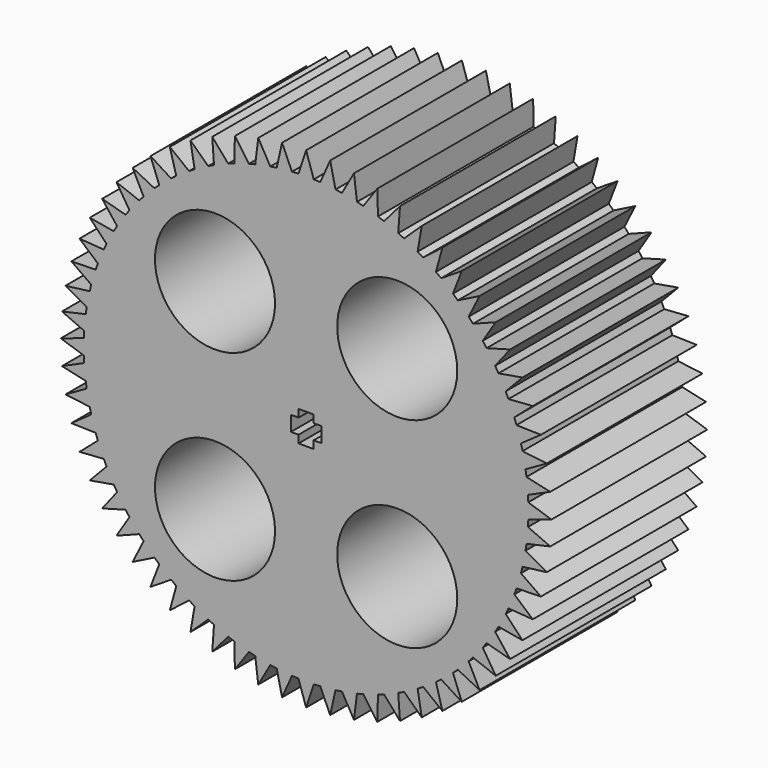
from build123d import *

# Parameters (mm, degrees)
F0_R     = 7.8312391684
F1_DEPTH = 7.0000114
F2_DEPTH = 25.4


with BuildPart() as f1:
    # F0 (on Front) → F1 (new body)
    with BuildSketch(Plane.XZ):
        with BuildLine():
            ThreePointArc((-1.00000054, 28.9827594773), (0, 29.000006), (1.00000054, 28.9827594773))
            Line((1.00000054, 28.9827594773), (0, 32))
            Line((0, 32), (-1.00000054, 28.9827594773))
        make_face()
        with BuildLine():
            ThreePointArc((1.8456219388, 28.9412167619), (2.8424976577, 28.8603630446), (3.8359924669, 28.7451823754))
            Line((3.8359924669, 28.7451823754), (3.1365484905, 31.8459112535))
            Line((3.1365484905, 31.8459112535), (1.8456219388, 28.9412167619))
        make_face()
        with BuildLine():
            ThreePointArc((4.6734700693, 28.6209543082), (5.657620509, 28.4427790164), (6.6350416894, 28.2307734535))
            Line((6.6350416894, 28.2307734535), (6.2428903045, 31.3851289729))
            Line((6.2428903045, 31.3851289729), (4.6734700693, 28.6209543082))
        make_face()
        with BuildLine():
            ThreePointArc((7.4563101283, 28.0250564187), (8.4182573821, 27.7512754779), (9.3701918333, 27.4444867507))
            Line((9.3701918333, 27.4444867507), (9.2891096721, 30.6220907434))
            Line((9.2891096721, 30.6220907434), (7.4563101283, 28.0250564187))
        make_face()
        with BuildLine():
            ThreePointArc((10.1673418448, 27.1592619158), (11.0978218347, 26.7925119861), (12.0151019076, 26.3938946378))
            Line((12.0151019076, 26.3938946378), (12.2458698357, 29.5641450404))
            Line((12.2458698357, 29.5641450404), (10.1673418448, 27.1592619158))
        make_face()
        with BuildLine():
            ThreePointArc((12.7804565012, 26.0319088739), (13.6705081963, 25.5757219576), (14.5442999824, 25.0891148912))
            Line((14.5442999824, 25.0891148912), (15.0846955784, 28.2214804591))
            Line((15.0846955784, 28.2214804591), (12.7804565012, 26.0319088739))
        make_face()
        with BuildLine():
            Line((28.9827594773, -1.00000054), (28.9827594773, 1.00000054))
            ThreePointArc((28.9827594773, 1.00000054), (28.9650742227, 1.4229628499), (28.9412167619, 1.8456219388))
            Line((28.9412167619, 1.8456219388), (28.7451823754, 3.8359924669))
            ThreePointArc((28.7451823754, 3.8359924669), (28.686124724, 4.2551846396), (28.6209543082, 4.6734700693))
            Line((28.6209543082, 4.6734700693), (28.2307734535, 6.6350416894))
            ThreePointArc((28.2307734535, 6.6350416894), (28.1309121628, 7.0464266751), (28.0250564187, 7.4563101283))
            Line((28.0250564187, 7.4563101283), (27.4444867507, 9.3701918333))
            ThreePointArc((27.4444867507, 9.3701918333), (27.3047835396, 9.7698077697), (27.1592619158, 10.1673418448))
            Line((27.1592619158, 10.1673418448), (26.3938946378, 12.0151019076))
            ThreePointArc((26.3938946378, 12.0151019076), (26.2156949245, 12.3991002748), (26.0319088739, 12.7804565012))
            Line((26.0319088739, 12.7804565012), (25.0891148912, 14.5442999824))
            ThreePointArc((25.0891148912, 14.5442999824), (24.8741348364, 14.9089826662), (24.6538543191, 15.2704883751))
            Line((24.6538543191, 15.2704883751), (23.542713253, 16.9334284977))
            ThreePointArc((23.542713253, 16.9334284977), (23.2930232322, 17.2752834045), (23.03836967, 17.6134570982))
            Line((23.03836967, 17.6134570982), (21.7695824165, 19.1594788397))
            ThreePointArc((21.7695824165, 19.1594788397), (21.487587081, 19.4752137199), (21.2010129269, 19.7867986009))
            Line((21.2010129269, 19.7867986009), (19.7867986009, 21.2010129269))
            ThreePointArc((19.7867986009, 21.2010129269), (19.4752137199, 21.487587081), (19.1594788397, 21.7695824165))
            Line((19.1594788397, 21.7695824165), (17.6134570982, 23.03836967))
            ThreePointArc((17.6134570982, 23.03836967), (17.2752834045, 23.2930232322), (16.9334284977, 23.542713253))
            Line((16.9334284977, 23.542713253), (15.2704883751, 24.6538543191))
            ThreePointArc((15.2704883751, 24.6538543191), (14.9089826662, 24.8741348364), (14.5442999824, 25.0891148912))
            Line((14.5442999824, 25.0891148912), (12.7804565012, 26.0319088739))
            ThreePointArc((12.7804565012, 26.0319088739), (12.3991002748, 26.2156949245), (12.0151019076, 26.3938946378))
            Line((12.0151019076, 26.3938946378), (10.1673418448, 27.1592619158))
            ThreePointArc((10.1673418448, 27.1592619158), (9.7698077697, 27.3047835396), (9.3701918333, 27.4444867507))
            Line((9.3701918333, 27.4444867507), (7.4563101283, 28.0250564187))
            ThreePointArc((7.4563101283, 28.0250564187), (7.0464266751, 28.1309121628), (6.6350416894, 28.2307734535))
            Line((6.6350416894, 28.2307734535), (4.6734700693, 28.6209543082))
            ThreePointArc((4.6734700693, 28.6209543082), (4.2551846396, 28.686124724), (3.8359924669, 28.7451823754))
            Line((3.8359924669, 28.7451823754), (1.8456219388, 28.9412167619))
            ThreePointArc((1.8456219388, 28.9412167619), (1.4229628499, 28.9650742227), (1.00000054, 28.9827594773))
            Line((1.00000054, 28.9827594773), (-1.00000054, 28.9827594773))
            ThreePointArc((-1.00000054, 28.9827594773), (-1.4229628499, 28.9650742227), (-1.8456219388, 28.9412167619))
            Line((-1.8456219388, 28.9412167619), (-3.8359924669, 28.7451823754))
            ThreePointArc((-3.8359924669, 28.7451823754), (-4.2551846396, 28.686124724), (-4.6734700693, 28.6209543082))
            Line((-4.6734700693, 28.6209543082), (-6.6350416894, 28.2307734535))
            ThreePointArc((-6.6350416894, 28.2307734535), (-7.0464266751, 28.1309121628), (-7.4563101283, 28.0250564187))
            Line((-7.4563101283, 28.0250564187), (-9.3701918333, 27.4444867507))
            ThreePointArc((-9.3701918333, 27.4444867507), (-9.7698077697, 27.3047835396), (-10.1673418448, 27.1592619158))
            Line((-10.1673418448, 27.1592619158), (-12.0151019076, 26.3938946378))
            ThreePointArc((-12.0151019076, 26.3938946378), (-12.3991002748, 26.2156949245), (-12.7804565012, 26.0319088739))
            Line((-12.7804565012, 26.0319088739), (-14.5442999824, 25.0891148912))
            ThreePointArc((-14.5442999824, 25.0891148912), (-14.9089826662, 24.8741348364), (-15.2704883751, 24.6538543191))
            Line((-15.2704883751, 24.6538543191), (-16.9334284977, 23.542713253))
            ThreePointArc((-16.9334284977, 23.542713253), (-17.2752834045, 23.2930232322), (-17.6134570982, 23.03836967))
            Line((-17.6134570982, 23.03836967), (-19.1594788397, 21.7695824165))
            ThreePointArc((-19.1594788397, 21.7695824165), (-19.4752137199, 21.487587081), (-19.7867986009, 21.2010129269))
            Line((-19.7867986009, 21.2010129269), (-21.2010129269, 19.7867986009))
            ThreePointArc((-21.2010129269, 19.7867986009), (-21.487587081, 19.4752137199), (-21.7695824165, 19.1594788397))
            Line((-21.7695824165, 19.1594788397), (-23.03836967, 17.6134570982))
            ThreePointArc((-23.03836967, 17.6134570982), (-23.2930232322, 17.2752834045), (-23.542713253, 16.9334284977))
            Line((-23.542713253, 16.9334284977), (-24.6538543191, 15.2704883751))
            ThreePointArc((-24.6538543191, 15.2704883751), (-24.8741348364, 14.9089826662), (-25.0891148912, 14.5442999824))
            Line((-25.0891148912, 14.5442999824), (-26.0319088739, 12.7804565012))
            ThreePointArc((-26.0319088739, 12.7804565012), (-26.2156949245, 12.3991002748), (-26.3938946378, 12.0151019076))
            Line((-26.3938946378, 12.0151019076), (-27.1592619158, 10.1673418448))
            ThreePointArc((-27.1592619158, 10.1673418448), (-27.3047835396, 9.7698077697), (-27.4444867507, 9.3701918333))
            Line((-27.4444867507, 9.3701918333), (-28.0250564187, 7.4563101283))
            ThreePointArc((-28.0250564187, 7.4563101283), (-28.1309121628, 7.0464266751), (-28.2307734535, 6.6350416894))
            Line((-28.2307734535, 6.6350416894), (-28.6209543082, 4.6734700693))
            ThreePointArc((-28.6209543082, 4.6734700693), (-28.686124724, 4.2551846396), (-28.7451823754, 3.8359924669))
            Line((-28.7451823754, 3.8359924669), (-28.9412167619, 1.8456219388))
            ThreePointArc((-28.9412167619, 1.8456219388), (-28.9650742227, 1.4229628499), (-28.9827594773, 1.00000054))
            Line((-28.9827594773, 1.00000054), (-28.9827594773, -1.00000054))
            ThreePointArc((-28.9827594773, -1.00000054), (-28.9650742227, -1.4229628499), (-28.9412167619, -1.8456219388))
            Line((-28.9412167619, -1.8456219388), (-28.7451823754, -3.8359924669))
            ThreePointArc((-28.7451823754, -3.8359924669), (-28.686124724, -4.2551846396), (-28.6209543082, -4.6734700693))
            Line((-28.6209543082, -4.6734700693), (-28.2307734535, -6.6350416894))
            ThreePointArc((-28.2307734535, -6.6350416894), (-28.1309121628, -7.0464266751), (-28.0250564187, -7.4563101283))
            Line((-28.0250564187, -7.4563101283), (-27.4444867507, -9.3701918333))
            ThreePointArc((-27.4444867507, -9.3701918333), (-27.3047835396, -9.7698077697), (-27.1592619158, -10.1673418448))
            Line((-27.1592619158, -10.1673418448), (-26.3938946378, -12.0151019076))
            ThreePointArc((-26.3938946378, -12.0151019076), (-26.2156949245, -12.3991002748), (-26.0319088739, -12.7804565012))
            Line((-26.0319088739, -12.7804565012), (-25.0891148912, -14.5442999824))
            ThreePointArc((-25.0891148912, -14.5442999824), (-24.8741348364, -14.9089826662), (-24.6538543191, -15.2704883751))
            Line((-24.6538543191, -15.2704883751), (-23.542713253, -16.9334284977))
            ThreePointArc((-23.542713253, -16.9334284977), (-23.2930232322, -17.2752834045), (-23.03836967, -17.6134570982))
            Line((-23.03836967, -17.6134570982), (-21.7695824165, -19.1594788397))
            ThreePointArc((-21.7695824165, -19.1594788397), (-21.487587081, -19.4752137199), (-21.2010129269, -19.7867986009))
            Line((-21.2010129269, -19.7867986009), (-19.7867986009, -21.2010129269))
            ThreePointArc((-19.7867986009, -21.2010129269), (-19.4752137199, -21.487587081), (-19.1594788397, -21.7695824165))
            Line((-19.1594788397, -21.7695824165), (-17.6134570982, -23.03836967))
            ThreePointArc((-17.6134570982, -23.03836967), (-17.2752834045, -23.2930232322), (-16.9334284977, -23.542713253))
            Line((-16.9334284977, -23.542713253), (-15.2704883751, -24.6538543191))
            ThreePointArc((-15.2704883751, -24.6538543191), (-14.9089826662, -24.8741348364), (-14.5442999824, -25.0891148912))
            Line((-14.5442999824, -25.0891148912), (-12.7804565012, -26.0319088739))
            ThreePointArc((-12.7804565012, -26.0319088739), (-12.3991002748, -26.2156949245), (-12.0151019076, -26.3938946378))
            Line((-12.0151019076, -26.3938946378), (-10.1673418448, -27.1592619158))
            ThreePointArc((-10.1673418448, -27.1592619158), (-9.7698077697, -27.3047835396), (-9.3701918333, -27.4444867507))
            Line((-9.3701918333, -27.4444867507), (-7.4563101283, -28.0250564187))
            ThreePointArc((-7.4563101283, -28.0250564187), (-7.0464266751, -28.1309121628), (-6.6350416894, -28.2307734535))
            Line((-6.6350416894, -28.2307734535), (-4.6734700693, -28.6209543082))
            ThreePointArc((-4.6734700693, -28.6209543082), (-4.2551846396, -28.686124724), (-3.8359924669, -28.7451823754))
            Line((-3.8359924669, -28.7451823754), (-1.8456219388, -28.9412167619))
            ThreePointArc((-1.8456219388, -28.9412167619), (-1.4229628499, -28.9650742227), (-1.00000054, -28.9827594773))
            Line((-1.00000054, -28.9827594773), (1.00000054, -28.9827594773))
            ThreePointArc((1.00000054, -28.9827594773), (1.4229628499, -28.9650742227), (1.8456219388, -28.9412167619))
            Line((1.8456219388, -28.9412167619), (3.8359924669, -28.7451823754))
            ThreePointArc((3.8359924669, -28.7451823754), (4.2551846396, -28.686124724), (4.6734700693, -28.6209543082))
            Line((4.6734700693, -28.6209543082), (6.6350416894, -28.2307734535))
            ThreePointArc((6.6350416894, -28.2307734535), (7.0464266751, -28.1309121628), (7.4563101283, -28.0250564187))
            Line((7.4563101283, -28.0250564187), (9.3701918333, -27.4444867507))
            ThreePointArc((9.3701918333, -27.4444867507), (9.7698077697, -27.3047835396), (10.1673418448, -27.1592619158))
            Line((10.1673418448, -27.1592619158), (12.0151019076, -26.3938946378))
            ThreePointArc((12.0151019076, -26.3938946378), (12.3991002748, -26.2156949245), (12.7804565012, -26.0319088739))
            Line((12.7804565012, -26.0319088739), (14.5442999824, -25.0891148912))
            ThreePointArc((14.5442999824, -25.0891148912), (14.9089826662, -24.8741348364), (15.2704883751, -24.6538543191))
            Line((15.2704883751, -24.6538543191), (16.9334284977, -23.542713253))
            ThreePointArc((16.9334284977, -23.542713253), (17.2752834045, -23.2930232322), (17.6134570982, -23.03836967))
            Line((17.6134570982, -23.03836967), (19.1594788397, -21.7695824165))
            ThreePointArc((19.1594788397, -21.7695824165), (19.4752137199, -21.487587081), (19.7867986009, -21.2010129269))
            Line((19.7867986009, -21.2010129269), (21.2010129269, -19.7867986009))
            ThreePointArc((21.2010129269, -19.7867986009), (21.487587081, -19.4752137199), (21.7695824165, -19.1594788397))
            Line((21.7695824165, -19.1594788397), (23.03836967, -17.6134570982))
            ThreePointArc((23.03836967, -17.6134570982), (23.2930232322, -17.2752834045), (23.542713253, -16.9334284977))
            Line((23.542713253, -16.9334284977), (24.6538543191, -15.2704883751))
            ThreePointArc((24.6538543191, -15.2704883751), (24.8741348364, -14.9089826662), (25.0891148912, -14.5442999824))
            Line((25.0891148912, -14.5442999824), (26.0319088739, -12.7804565012))
            ThreePointArc((26.0319088739, -12.7804565012), (26.2156949245, -12.3991002748), (26.3938946378, -12.0151019076))
            Line((26.3938946378, -12.0151019076), (27.1592619158, -10.1673418448))
            ThreePointArc((27.1592619158, -10.1673418448), (27.3047835396, -9.7698077697), (27.4444867507, -9.3701918333))
            Line((27.4444867507, -9.3701918333), (28.0250564187, -7.4563101283))
            ThreePointArc((28.0250564187, -7.4563101283), (28.1309121628, -7.0464266751), (28.2307734535, -6.6350416894))
            Line((28.2307734535, -6.6350416894), (28.6209543082, -4.6734700693))
            ThreePointArc((28.6209543082, -4.6734700693), (28.686124724, -4.2551846396), (28.7451823754, -3.8359924669))
            Line((28.7451823754, -3.8359924669), (28.9412167619, -1.8456219388))
            ThreePointArc((28.9412167619, -1.8456219388), (28.9650742227, -1.4229628499), (28.9827594773, -1.00000054))
        make_face()
        with Locations((-11.8841798976, -13.0854817107)):
            Circle(F0_R, mode=Mode.SUBTRACT)
        with Locations((11.8841798976, -13.0854817107)):
            Circle(F0_R, mode=Mode.SUBTRACT)
        with Locations((-11.8841798976, 13.0854817107)):
            Circle(F0_R, mode=Mode.SUBTRACT)
        Polygon((-0.98349054, 0.98349054), (-0.98349054, 1.98349108), (0.98349054, 1.98349108), (0.98349054, 0.98349054), (1.98349108, 0.98349054), (1.98349108, -0.98349054), (0.98349054, -0.98349054), (0.98349054, -1.98349108), (-0.98349054, -1.98349108), (-0.98349054, -0.98349054), (-1.98349108, -0.98349054), (-1.98349108, 0.98349054), align=None, mode=Mode.SUBTRACT)
        with Locations((11.8841798976, 13.0854817107)):
            Circle(F0_R, mode=Mode.SUBTRACT)
        with BuildLine():
            ThreePointArc((15.2704883751, 24.6538543191), (16.111540091, 24.1126237456), (16.9334284977, 23.542713253))
            Line((16.9334284977, 23.542713253), (17.7782474566, 26.6070275937))
            Line((17.7782474566, 26.6070275937), (15.2704883751, 24.6538543191))
        make_face()
        with BuildLine():
            ThreePointArc((17.6134570982, 23.03836967), (18.3974090471, 22.4173077856), (19.1594788397, 21.7695824165))
            Line((19.1594788397, 21.7695824165), (20.3005850932, 24.7363345076))
            Line((20.3005850932, 24.7363345076), (17.6134570982, 23.03836967))
        make_face()
        with BuildLine():
            ThreePointArc((19.7867986009, 21.2010129269), (20.5061008971, 20.5061008971), (21.2010129269, 19.7867986009))
            Line((21.2010129269, 19.7867986009), (22.627416998, 22.627416998))
            Line((22.627416998, 22.627416998), (19.7867986009, 21.2010129269))
        make_face()
        with BuildLine():
            ThreePointArc((21.7695824165, 19.1594788397), (22.4173077856, 18.3974090471), (23.03836967, 17.6134570982))
            Line((23.03836967, 17.6134570982), (24.7363345076, 20.3005850932))
            Line((24.7363345076, 20.3005850932), (21.7695824165, 19.1594788397))
        make_face()
        with BuildLine():
            ThreePointArc((23.542713253, 16.9334284977), (24.1126237456, 16.111540091), (24.6538543191, 15.2704883751))
            Line((24.6538543191, 15.2704883751), (26.6070275937, 17.7782474566))
            Line((26.6070275937, 17.7782474566), (23.542713253, 16.9334284977))
        make_face()
        with BuildLine():
            ThreePointArc((25.0891148912, 14.5442999824), (25.5757219576, 13.6705081963), (26.0319088739, 12.7804565012))
            Line((26.0319088739, 12.7804565012), (28.2214804591, 15.0846955784))
            Line((28.2214804591, 15.0846955784), (25.0891148912, 14.5442999824))
        make_face()
        with BuildLine():
            ThreePointArc((26.3938946378, 12.0151019076), (26.7925119861, 11.0978218347), (27.1592619158, 10.1673418448))
            Line((27.1592619158, 10.1673418448), (29.5641450404, 12.2458698357))
            Line((29.5641450404, 12.2458698357), (26.3938946378, 12.0151019076))
        make_face()
        with BuildLine():
            ThreePointArc((27.4444867507, 9.3701918333), (27.7512754779, 8.4182573821), (28.0250564187, 7.4563101283))
            Line((28.0250564187, 7.4563101283), (30.6220907434, 9.2891096721))
            Line((30.6220907434, 9.2891096721), (27.4444867507, 9.3701918333))
        make_face()
        with BuildLine():
            ThreePointArc((28.2307734535, 6.6350416894), (28.4427790164, 5.657620509), (28.6209543082, 4.6734700693))
            Line((28.6209543082, 4.6734700693), (31.3851289729, 6.2428903045))
            Line((31.3851289729, 6.2428903045), (28.2307734535, 6.6350416894))
        make_face()
        with BuildLine():
            ThreePointArc((28.7451823754, 3.8359924669), (28.8603630446, 2.8424976577), (28.9412167619, 1.8456219388))
            Line((28.9412167619, 1.8456219388), (31.8459112535, 3.1365484905))
            Line((31.8459112535, 3.1365484905), (28.7451823754, 3.8359924669))
        make_face()
        with BuildLine():
            ThreePointArc((28.9827594773, 1.00000054), (28.9956940488, 0.5000746251), (29.000006, 0))
            ThreePointArc((29.000006, 0), (28.9956940488, -0.5000746251), (28.9827594773, -1.00000054))
            Line((28.9827594773, -1.00000054), (32, 0))
            Line((32, 0), (28.9827594773, 1.00000054))
        make_face()
        with BuildLine():
            Line((31.8459112535, -3.1365484905), (28.9412167619, -1.8456219388))
            ThreePointArc((28.9412167619, -1.8456219388), (28.8603630446, -2.8424976577), (28.7451823754, -3.8359924669))
            Line((28.7451823754, -3.8359924669), (31.8459112535, -3.1365484905))
        make_face()
        with BuildLine():
            Line((31.3851289729, -6.2428903045), (28.6209543082, -4.6734700693))
            ThreePointArc((28.6209543082, -4.6734700693), (28.4427790164, -5.657620509), (28.2307734535, -6.6350416894))
            Line((28.2307734535, -6.6350416894), (31.3851289729, -6.2428903045))
        make_face()
        with BuildLine():
            Line((30.6220907434, -9.2891096721), (28.0250564187, -7.4563101283))
            ThreePointArc((28.0250564187, -7.4563101283), (27.7512754779, -8.4182573821), (27.4444867507, -9.3701918333))
            Line((27.4444867507, -9.3701918333), (30.6220907434, -9.2891096721))
        make_face()
        with BuildLine():
            Line((29.5641450404, -12.2458698357), (27.1592619158, -10.1673418448))
            ThreePointArc((27.1592619158, -10.1673418448), (26.7925119861, -11.0978218347), (26.3938946378, -12.0151019076))
            Line((26.3938946378, -12.0151019076), (29.5641450404, -12.2458698357))
        make_face()
        with BuildLine():
            Line((26.6070275937, -17.7782474566), (24.6538543191, -15.2704883751))
            ThreePointArc((24.6538543191, -15.2704883751), (24.1126237456, -16.111540091), (23.542713253, -16.9334284977))
            Line((23.542713253, -16.9334284977), (26.6070275937, -17.7782474566))
        make_face()
        with BuildLine():
            Line((28.2214804591, -15.0846955784), (26.0319088739, -12.7804565012))
            ThreePointArc((26.0319088739, -12.7804565012), (25.5757219576, -13.6705081963), (25.0891148912, -14.5442999824))
            Line((25.0891148912, -14.5442999824), (28.2214804591, -15.0846955784))
        make_face()
        with BuildLine():
            Line((24.7363345076, -20.3005850932), (23.03836967, -17.6134570982))
            ThreePointArc((23.03836967, -17.6134570982), (22.4173077856, -18.3974090471), (21.7695824165, -19.1594788397))
            Line((21.7695824165, -19.1594788397), (24.7363345076, -20.3005850932))
        make_face()
        with BuildLine():
            Line((22.627416998, -22.627416998), (21.2010129269, -19.7867986009))
            ThreePointArc((21.2010129269, -19.7867986009), (20.5061008971, -20.5061008971), (19.7867986009, -21.2010129269))
            Line((19.7867986009, -21.2010129269), (22.627416998, -22.627416998))
        make_face()
        with BuildLine():
            Line((20.3005850932, -24.7363345076), (19.1594788397, -21.7695824165))
            ThreePointArc((19.1594788397, -21.7695824165), (18.3974090471, -22.4173077856), (17.6134570982, -23.03836967))
            Line((17.6134570982, -23.03836967), (20.3005850932, -24.7363345076))
        make_face()
        with BuildLine():
            Line((17.7782474566, -26.6070275937), (16.9334284977, -23.542713253))
            ThreePointArc((16.9334284977, -23.542713253), (16.111540091, -24.1126237456), (15.2704883751, -24.6538543191))
            Line((15.2704883751, -24.6538543191), (17.7782474566, -26.6070275937))
        make_face()
        with BuildLine():
            Line((15.0846955784, -28.2214804591), (14.5442999824, -25.0891148912))
            ThreePointArc((14.5442999824, -25.0891148912), (13.6705081963, -25.5757219576), (12.7804565012, -26.0319088739))
            Line((12.7804565012, -26.0319088739), (15.0846955784, -28.2214804591))
        make_face()
        with BuildLine():
            Line((12.2458698357, -29.5641450404), (12.0151019076, -26.3938946378))
            ThreePointArc((12.0151019076, -26.3938946378), (11.0978218347, -26.7925119861), (10.1673418448, -27.1592619158))
            Line((10.1673418448, -27.1592619158), (12.2458698357, -29.5641450404))
        make_face()
        with BuildLine():
            Line((9.2891096721, -30.6220907434), (9.3701918333, -27.4444867507))
            ThreePointArc((9.3701918333, -27.4444867507), (8.4182573821, -27.7512754779), (7.4563101283, -28.0250564187))
            Line((7.4563101283, -28.0250564187), (9.2891096721, -30.6220907434))
        make_face()
        with BuildLine():
            Line((6.2428903045, -31.3851289729), (6.6350416894, -28.2307734535))
            ThreePointArc((6.6350416894, -28.2307734535), (5.657620509, -28.4427790164), (4.6734700693, -28.6209543082))
            Line((4.6734700693, -28.6209543082), (6.2428903045, -31.3851289729))
        make_face()
        with BuildLine():
            Line((3.1365484905, -31.8459112535), (3.8359924669, -28.7451823754))
            ThreePointArc((3.8359924669, -28.7451823754), (2.8424976577, -28.8603630446), (1.8456219388, -28.9412167619))
            Line((1.8456219388, -28.9412167619), (3.1365484905, -31.8459112535))
        make_face()
        with BuildLine():
            Line((0, -32), (1.00000054, -28.9827594773))
            ThreePointArc((1.00000054, -28.9827594773), (0, -29.000006), (-1.00000054, -28.9827594773))
            Line((-1.00000054, -28.9827594773), (0, -32))
        make_face()
        with BuildLine():
            Line((-3.1365484905, -31.8459112535), (-1.8456219388, -28.9412167619))
            ThreePointArc((-1.8456219388, -28.9412167619), (-2.8424976577, -28.8603630446), (-3.8359924669, -28.7451823754))
            Line((-3.8359924669, -28.7451823754), (-3.1365484905, -31.8459112535))
        make_face()
        with BuildLine():
            Line((-6.2428903045, -31.3851289729), (-4.6734700693, -28.6209543082))
            ThreePointArc((-4.6734700693, -28.6209543082), (-5.657620509, -28.4427790164), (-6.6350416894, -28.2307734535))
            Line((-6.6350416894, -28.2307734535), (-6.2428903045, -31.3851289729))
        make_face()
        with BuildLine():
            Line((-9.2891096721, -30.6220907434), (-7.4563101283, -28.0250564187))
            ThreePointArc((-7.4563101283, -28.0250564187), (-8.4182573821, -27.7512754779), (-9.3701918333, -27.4444867507))
            Line((-9.3701918333, -27.4444867507), (-9.2891096721, -30.6220907434))
        make_face()
        with BuildLine():
            Line((-12.2458698357, -29.5641450404), (-10.1673418448, -27.1592619158))
            ThreePointArc((-10.1673418448, -27.1592619158), (-11.0978218347, -26.7925119861), (-12.0151019076, -26.3938946378))
            Line((-12.0151019076, -26.3938946378), (-12.2458698357, -29.5641450404))
        make_face()
        with BuildLine():
            Line((-15.0846955784, -28.2214804591), (-12.7804565012, -26.0319088739))
            ThreePointArc((-12.7804565012, -26.0319088739), (-13.6705081963, -25.5757219576), (-14.5442999824, -25.0891148912))
            Line((-14.5442999824, -25.0891148912), (-15.0846955784, -28.2214804591))
        make_face()
        with BuildLine():
            Line((-17.7782474566, -26.6070275937), (-15.2704883751, -24.6538543191))
            ThreePointArc((-15.2704883751, -24.6538543191), (-16.111540091, -24.1126237456), (-16.9334284977, -23.542713253))
            Line((-16.9334284977, -23.542713253), (-17.7782474566, -26.6070275937))
        make_face()
        with BuildLine():
            Line((-20.3005850932, -24.7363345076), (-17.6134570982, -23.03836967))
            ThreePointArc((-17.6134570982, -23.03836967), (-18.3974090471, -22.4173077856), (-19.1594788397, -21.7695824165))
            Line((-19.1594788397, -21.7695824165), (-20.3005850932, -24.7363345076))
        make_face()
        with BuildLine():
            Line((-22.627416998, -22.627416998), (-19.7867986009, -21.2010129269))
            ThreePointArc((-19.7867986009, -21.2010129269), (-20.5061008971, -20.5061008971), (-21.2010129269, -19.7867986009))
            Line((-21.2010129269, -19.7867986009), (-22.627416998, -22.627416998))
        make_face()
        with BuildLine():
            Line((-24.7363345076, -20.3005850932), (-21.7695824165, -19.1594788397))
            ThreePointArc((-21.7695824165, -19.1594788397), (-22.4173077856, -18.3974090471), (-23.03836967, -17.6134570982))
            Line((-23.03836967, -17.6134570982), (-24.7363345076, -20.3005850932))
        make_face()
        with BuildLine():
            Line((-26.6070275937, -17.7782474566), (-23.542713253, -16.9334284977))
            ThreePointArc((-23.542713253, -16.9334284977), (-24.1126237456, -16.111540091), (-24.6538543191, -15.2704883751))
            Line((-24.6538543191, -15.2704883751), (-26.6070275937, -17.7782474566))
        make_face()
        with BuildLine():
            Line((-28.2214804591, -15.0846955784), (-25.0891148912, -14.5442999824))
            ThreePointArc((-25.0891148912, -14.5442999824), (-25.5757219576, -13.6705081963), (-26.0319088739, -12.7804565012))
            Line((-26.0319088739, -12.7804565012), (-28.2214804591, -15.0846955784))
        make_face()
        with BuildLine():
            Line((-29.5641450404, -12.2458698357), (-26.3938946378, -12.0151019076))
            ThreePointArc((-26.3938946378, -12.0151019076), (-26.7925119861, -11.0978218347), (-27.1592619158, -10.1673418448))
            Line((-27.1592619158, -10.1673418448), (-29.5641450404, -12.2458698357))
        make_face()
        with BuildLine():
            Line((-30.6220907434, -9.2891096721), (-27.4444867507, -9.3701918333))
            ThreePointArc((-27.4444867507, -9.3701918333), (-27.7512754779, -8.4182573821), (-28.0250564187, -7.4563101283))
            Line((-28.0250564187, -7.4563101283), (-30.6220907434, -9.2891096721))
        make_face()
        with BuildLine():
            Line((-31.3851289729, -6.2428903045), (-28.2307734535, -6.6350416894))
            ThreePointArc((-28.2307734535, -6.6350416894), (-28.4427790164, -5.657620509), (-28.6209543082, -4.6734700693))
            Line((-28.6209543082, -4.6734700693), (-31.3851289729, -6.2428903045))
        make_face()
        with BuildLine():
            Line((-31.8459112535, -3.1365484905), (-28.7451823754, -3.8359924669))
            ThreePointArc((-28.7451823754, -3.8359924669), (-28.8603630446, -2.8424976577), (-28.9412167619, -1.8456219388))
            Line((-28.9412167619, -1.8456219388), (-31.8459112535, -3.1365484905))
        make_face()
        with BuildLine():
            ThreePointArc((-28.9412167619, 1.8456219388), (-28.8603630446, 2.8424976577), (-28.7451823754, 3.8359924669))
            Line((-28.7451823754, 3.8359924669), (-31.8459112535, 3.1365484905))
            Line((-31.8459112535, 3.1365484905), (-28.9412167619, 1.8456219388))
        make_face()
        with BuildLine():
            ThreePointArc((-28.9827594773, -1.00000054), (-29.000006, 0), (-28.9827594773, 1.00000054))
            Line((-28.9827594773, 1.00000054), (-32, 0))
            Line((-32, 0), (-28.9827594773, -1.00000054))
        make_face()
        with BuildLine():
            ThreePointArc((-28.6209543082, 4.6734700693), (-28.4427790164, 5.657620509), (-28.2307734535, 6.6350416894))
            Line((-28.2307734535, 6.6350416894), (-31.3851289729, 6.2428903045))
            Line((-31.3851289729, 6.2428903045), (-28.6209543082, 4.6734700693))
        make_face()
        with BuildLine():
            ThreePointArc((-28.0250564187, 7.4563101283), (-27.7512754779, 8.4182573821), (-27.4444867507, 9.3701918333))
            Line((-27.4444867507, 9.3701918333), (-30.6220907434, 9.2891096721))
            Line((-30.6220907434, 9.2891096721), (-28.0250564187, 7.4563101283))
        make_face()
        with BuildLine():
            ThreePointArc((-27.1592619158, 10.1673418448), (-26.7925119861, 11.0978218347), (-26.3938946378, 12.0151019076))
            Line((-26.3938946378, 12.0151019076), (-29.5641450404, 12.2458698357))
            Line((-29.5641450404, 12.2458698357), (-27.1592619158, 10.1673418448))
        make_face()
        with BuildLine():
            ThreePointArc((-26.0319088739, 12.7804565012), (-25.5757219576, 13.6705081963), (-25.0891148912, 14.5442999824))
            Line((-25.0891148912, 14.5442999824), (-28.2214804591, 15.0846955784))
            Line((-28.2214804591, 15.0846955784), (-26.0319088739, 12.7804565012))
        make_face()
        with BuildLine():
            ThreePointArc((-24.6538543191, 15.2704883751), (-24.1126237456, 16.111540091), (-23.542713253, 16.9334284977))
            Line((-23.542713253, 16.9334284977), (-26.6070275937, 17.7782474566))
            Line((-26.6070275937, 17.7782474566), (-24.6538543191, 15.2704883751))
        make_face()
        with BuildLine():
            ThreePointArc((-23.03836967, 17.6134570982), (-22.4173077856, 18.3974090471), (-21.7695824165, 19.1594788397))
            Line((-21.7695824165, 19.1594788397), (-24.7363345076, 20.3005850932))
            Line((-24.7363345076, 20.3005850932), (-23.03836967, 17.6134570982))
        make_face()
        with BuildLine():
            ThreePointArc((-21.2010129269, 19.7867986009), (-20.5061008971, 20.5061008971), (-19.7867986009, 21.2010129269))
            Line((-19.7867986009, 21.2010129269), (-22.627416998, 22.627416998))
            Line((-22.627416998, 22.627416998), (-21.2010129269, 19.7867986009))
        make_face()
        with BuildLine():
            ThreePointArc((-19.1594788397, 21.7695824165), (-18.3974090471, 22.4173077856), (-17.6134570982, 23.03836967))
            Line((-17.6134570982, 23.03836967), (-20.3005850932, 24.7363345076))
            Line((-20.3005850932, 24.7363345076), (-19.1594788397, 21.7695824165))
        make_face()
        with BuildLine():
            ThreePointArc((-16.9334284977, 23.542713253), (-16.111540091, 24.1126237456), (-15.2704883751, 24.6538543191))
            Line((-15.2704883751, 24.6538543191), (-17.7782474566, 26.6070275937))
            Line((-17.7782474566, 26.6070275937), (-16.9334284977, 23.542713253))
        make_face()
        with BuildLine():
            ThreePointArc((-14.5442999824, 25.0891148912), (-13.6705081963, 25.5757219576), (-12.7804565012, 26.0319088739))
            Line((-12.7804565012, 26.0319088739), (-15.0846955784, 28.2214804591))
            Line((-15.0846955784, 28.2214804591), (-14.5442999824, 25.0891148912))
        make_face()
        with BuildLine():
            ThreePointArc((-12.0151019076, 26.3938946378), (-11.0978218347, 26.7925119861), (-10.1673418448, 27.1592619158))
            Line((-10.1673418448, 27.1592619158), (-12.2458698357, 29.5641450404))
            Line((-12.2458698357, 29.5641450404), (-12.0151019076, 26.3938946378))
        make_face()
        with BuildLine():
            ThreePointArc((-9.3701918333, 27.4444867507), (-8.4182573821, 27.7512754779), (-7.4563101283, 28.0250564187))
            Line((-7.4563101283, 28.0250564187), (-9.2891096721, 30.6220907434))
            Line((-9.2891096721, 30.6220907434), (-9.3701918333, 27.4444867507))
        make_face()
        with BuildLine():
            ThreePointArc((-6.6350416894, 28.2307734535), (-5.657620509, 28.4427790164), (-4.6734700693, 28.6209543082))
            Line((-4.6734700693, 28.6209543082), (-6.2428903045, 31.3851289729))
            Line((-6.2428903045, 31.3851289729), (-6.6350416894, 28.2307734535))
        make_face()
        with BuildLine():
            ThreePointArc((-3.8359924669, 28.7451823754), (-2.8424976577, 28.8603630446), (-1.8456219388, 28.9412167619))
            Line((-1.8456219388, 28.9412167619), (-3.1365484905, 31.8459112535))
            Line((-3.1365484905, 31.8459112535), (-3.8359924669, 28.7451823754))
        make_face()
    extrude(amount=F1_DEPTH)


with BuildPart() as f2:
    # F0 (on Front) → F2 (new body)
    with BuildSketch(Plane.XZ):
        with BuildLine():
            ThreePointArc((28.9827594773, -1.00000054), (28.9956940488, -0.5000746251), (29.000006, 0))
            ThreePointArc((29.000006, 0), (28.9956940488, 0.5000746251), (28.9827594773, 1.00000054))
            Line((28.9827594773, 1.00000054), (28.9827594773, -1.00000054))
        make_face()
        with BuildLine():
            ThreePointArc((28.9827594773, 1.00000054), (28.9956940488, 0.5000746251), (29.000006, 0))
            ThreePointArc((29.000006, 0), (28.9956940488, -0.5000746251), (28.9827594773, -1.00000054))
            Line((28.9827594773, -1.00000054), (32, 0))
            Line((32, 0), (28.9827594773, 1.00000054))
        make_face()
        with BuildLine():
            Line((28.9827594773, -1.00000054), (28.9827594773, 1.00000054))
            ThreePointArc((28.9827594773, 1.00000054), (28.9650742227, 1.4229628499), (28.9412167619, 1.8456219388))
            Line((28.9412167619, 1.8456219388), (28.7451823754, 3.8359924669))
            ThreePointArc((28.7451823754, 3.8359924669), (28.686124724, 4.2551846396), (28.6209543082, 4.6734700693))
            Line((28.6209543082, 4.6734700693), (28.2307734535, 6.6350416894))
            ThreePointArc((28.2307734535, 6.6350416894), (28.1309121628, 7.0464266751), (28.0250564187, 7.4563101283))
            Line((28.0250564187, 7.4563101283), (27.4444867507, 9.3701918333))
            ThreePointArc((27.4444867507, 9.3701918333), (27.3047835396, 9.7698077697), (27.1592619158, 10.1673418448))
            Line((27.1592619158, 10.1673418448), (26.3938946378, 12.0151019076))
            ThreePointArc((26.3938946378, 12.0151019076), (26.2156949245, 12.3991002748), (26.0319088739, 12.7804565012))
            Line((26.0319088739, 12.7804565012), (25.0891148912, 14.5442999824))
            ThreePointArc((25.0891148912, 14.5442999824), (24.8741348364, 14.9089826662), (24.6538543191, 15.2704883751))
            Line((24.6538543191, 15.2704883751), (23.542713253, 16.9334284977))
            ThreePointArc((23.542713253, 16.9334284977), (23.2930232322, 17.2752834045), (23.03836967, 17.6134570982))
            Line((23.03836967, 17.6134570982), (21.7695824165, 19.1594788397))
            ThreePointArc((21.7695824165, 19.1594788397), (21.487587081, 19.4752137199), (21.2010129269, 19.7867986009))
            Line((21.2010129269, 19.7867986009), (19.7867986009, 21.2010129269))
            ThreePointArc((19.7867986009, 21.2010129269), (19.4752137199, 21.487587081), (19.1594788397, 21.7695824165))
            Line((19.1594788397, 21.7695824165), (17.6134570982, 23.03836967))
            ThreePointArc((17.6134570982, 23.03836967), (17.2752834045, 23.2930232322), (16.9334284977, 23.542713253))
            Line((16.9334284977, 23.542713253), (15.2704883751, 24.6538543191))
            ThreePointArc((15.2704883751, 24.6538543191), (14.9089826662, 24.8741348364), (14.5442999824, 25.0891148912))
            Line((14.5442999824, 25.0891148912), (12.7804565012, 26.0319088739))
            ThreePointArc((12.7804565012, 26.0319088739), (12.3991002748, 26.2156949245), (12.0151019076, 26.3938946378))
            Line((12.0151019076, 26.3938946378), (10.1673418448, 27.1592619158))
            ThreePointArc((10.1673418448, 27.1592619158), (9.7698077697, 27.3047835396), (9.3701918333, 27.4444867507))
            Line((9.3701918333, 27.4444867507), (7.4563101283, 28.0250564187))
            ThreePointArc((7.4563101283, 28.0250564187), (7.0464266751, 28.1309121628), (6.6350416894, 28.2307734535))
            Line((6.6350416894, 28.2307734535), (4.6734700693, 28.6209543082))
            ThreePointArc((4.6734700693, 28.6209543082), (4.2551846396, 28.686124724), (3.8359924669, 28.7451823754))
            Line((3.8359924669, 28.7451823754), (1.8456219388, 28.9412167619))
            ThreePointArc((1.8456219388, 28.9412167619), (1.4229628499, 28.9650742227), (1.00000054, 28.9827594773))
            Line((1.00000054, 28.9827594773), (-1.00000054, 28.9827594773))
            ThreePointArc((-1.00000054, 28.9827594773), (-1.4229628499, 28.9650742227), (-1.8456219388, 28.9412167619))
            Line((-1.8456219388, 28.9412167619), (-3.8359924669, 28.7451823754))
            ThreePointArc((-3.8359924669, 28.7451823754), (-4.2551846396, 28.686124724), (-4.6734700693, 28.6209543082))
            Line((-4.6734700693, 28.6209543082), (-6.6350416894, 28.2307734535))
            ThreePointArc((-6.6350416894, 28.2307734535), (-7.0464266751, 28.1309121628), (-7.4563101283, 28.0250564187))
            Line((-7.4563101283, 28.0250564187), (-9.3701918333, 27.4444867507))
            ThreePointArc((-9.3701918333, 27.4444867507), (-9.7698077697, 27.3047835396), (-10.1673418448, 27.1592619158))
            Line((-10.1673418448, 27.1592619158), (-12.0151019076, 26.3938946378))
            ThreePointArc((-12.0151019076, 26.3938946378), (-12.3991002748, 26.2156949245), (-12.7804565012, 26.0319088739))
            Line((-12.7804565012, 26.0319088739), (-14.5442999824, 25.0891148912))
            ThreePointArc((-14.5442999824, 25.0891148912), (-14.9089826662, 24.8741348364), (-15.2704883751, 24.6538543191))
            Line((-15.2704883751, 24.6538543191), (-16.9334284977, 23.542713253))
            ThreePointArc((-16.9334284977, 23.542713253), (-17.2752834045, 23.2930232322), (-17.6134570982, 23.03836967))
            Line((-17.6134570982, 23.03836967), (-19.1594788397, 21.7695824165))
            ThreePointArc((-19.1594788397, 21.7695824165), (-19.4752137199, 21.487587081), (-19.7867986009, 21.2010129269))
            Line((-19.7867986009, 21.2010129269), (-21.2010129269, 19.7867986009))
            ThreePointArc((-21.2010129269, 19.7867986009), (-21.487587081, 19.4752137199), (-21.7695824165, 19.1594788397))
            Line((-21.7695824165, 19.1594788397), (-23.03836967, 17.6134570982))
            ThreePointArc((-23.03836967, 17.6134570982), (-23.2930232322, 17.2752834045), (-23.542713253, 16.9334284977))
            Line((-23.542713253, 16.9334284977), (-24.6538543191, 15.2704883751))
            ThreePointArc((-24.6538543191, 15.2704883751), (-24.8741348364, 14.9089826662), (-25.0891148912, 14.5442999824))
            Line((-25.0891148912, 14.5442999824), (-26.0319088739, 12.7804565012))
            ThreePointArc((-26.0319088739, 12.7804565012), (-26.2156949245, 12.3991002748), (-26.3938946378, 12.0151019076))
            Line((-26.3938946378, 12.0151019076), (-27.1592619158, 10.1673418448))
            ThreePointArc((-27.1592619158, 10.1673418448), (-27.3047835396, 9.7698077697), (-27.4444867507, 9.3701918333))
            Line((-27.4444867507, 9.3701918333), (-28.0250564187, 7.4563101283))
            ThreePointArc((-28.0250564187, 7.4563101283), (-28.1309121628, 7.0464266751), (-28.2307734535, 6.6350416894))
            Line((-28.2307734535, 6.6350416894), (-28.6209543082, 4.6734700693))
            ThreePointArc((-28.6209543082, 4.6734700693), (-28.686124724, 4.2551846396), (-28.7451823754, 3.8359924669))
            Line((-28.7451823754, 3.8359924669), (-28.9412167619, 1.8456219388))
            ThreePointArc((-28.9412167619, 1.8456219388), (-28.9650742227, 1.4229628499), (-28.9827594773, 1.00000054))
            Line((-28.9827594773, 1.00000054), (-28.9827594773, -1.00000054))
            ThreePointArc((-28.9827594773, -1.00000054), (-28.9650742227, -1.4229628499), (-28.9412167619, -1.8456219388))
            Line((-28.9412167619, -1.8456219388), (-28.7451823754, -3.8359924669))
            ThreePointArc((-28.7451823754, -3.8359924669), (-28.686124724, -4.2551846396), (-28.6209543082, -4.6734700693))
            Line((-28.6209543082, -4.6734700693), (-28.2307734535, -6.6350416894))
            ThreePointArc((-28.2307734535, -6.6350416894), (-28.1309121628, -7.0464266751), (-28.0250564187, -7.4563101283))
            Line((-28.0250564187, -7.4563101283), (-27.4444867507, -9.3701918333))
            ThreePointArc((-27.4444867507, -9.3701918333), (-27.3047835396, -9.7698077697), (-27.1592619158, -10.1673418448))
            Line((-27.1592619158, -10.1673418448), (-26.3938946378, -12.0151019076))
            ThreePointArc((-26.3938946378, -12.0151019076), (-26.2156949245, -12.3991002748), (-26.0319088739, -12.7804565012))
            Line((-26.0319088739, -12.7804565012), (-25.0891148912, -14.5442999824))
            ThreePointArc((-25.0891148912, -14.5442999824), (-24.8741348364, -14.9089826662), (-24.6538543191, -15.2704883751))
            Line((-24.6538543191, -15.2704883751), (-23.542713253, -16.9334284977))
            ThreePointArc((-23.542713253, -16.9334284977), (-23.2930232322, -17.2752834045), (-23.03836967, -17.6134570982))
            Line((-23.03836967, -17.6134570982), (-21.7695824165, -19.1594788397))
            ThreePointArc((-21.7695824165, -19.1594788397), (-21.487587081, -19.4752137199), (-21.2010129269, -19.7867986009))
            Line((-21.2010129269, -19.7867986009), (-19.7867986009, -21.2010129269))
            ThreePointArc((-19.7867986009, -21.2010129269), (-19.4752137199, -21.487587081), (-19.1594788397, -21.7695824165))
            Line((-19.1594788397, -21.7695824165), (-17.6134570982, -23.03836967))
            ThreePointArc((-17.6134570982, -23.03836967), (-17.2752834045, -23.2930232322), (-16.9334284977, -23.542713253))
            Line((-16.9334284977, -23.542713253), (-15.2704883751, -24.6538543191))
            ThreePointArc((-15.2704883751, -24.6538543191), (-14.9089826662, -24.8741348364), (-14.5442999824, -25.0891148912))
            Line((-14.5442999824, -25.0891148912), (-12.7804565012, -26.0319088739))
            ThreePointArc((-12.7804565012, -26.0319088739), (-12.3991002748, -26.2156949245), (-12.0151019076, -26.3938946378))
            Line((-12.0151019076, -26.3938946378), (-10.1673418448, -27.1592619158))
            ThreePointArc((-10.1673418448, -27.1592619158), (-9.7698077697, -27.3047835396), (-9.3701918333, -27.4444867507))
            Line((-9.3701918333, -27.4444867507), (-7.4563101283, -28.0250564187))
            ThreePointArc((-7.4563101283, -28.0250564187), (-7.0464266751, -28.1309121628), (-6.6350416894, -28.2307734535))
            Line((-6.6350416894, -28.2307734535), (-4.6734700693, -28.6209543082))
            ThreePointArc((-4.6734700693, -28.6209543082), (-4.2551846396, -28.686124724), (-3.8359924669, -28.7451823754))
            Line((-3.8359924669, -28.7451823754), (-1.8456219388, -28.9412167619))
            ThreePointArc((-1.8456219388, -28.9412167619), (-1.4229628499, -28.9650742227), (-1.00000054, -28.9827594773))
            Line((-1.00000054, -28.9827594773), (1.00000054, -28.9827594773))
            ThreePointArc((1.00000054, -28.9827594773), (1.4229628499, -28.9650742227), (1.8456219388, -28.9412167619))
            Line((1.8456219388, -28.9412167619), (3.8359924669, -28.7451823754))
            ThreePointArc((3.8359924669, -28.7451823754), (4.2551846396, -28.686124724), (4.6734700693, -28.6209543082))
            Line((4.6734700693, -28.6209543082), (6.6350416894, -28.2307734535))
            ThreePointArc((6.6350416894, -28.2307734535), (7.0464266751, -28.1309121628), (7.4563101283, -28.0250564187))
            Line((7.4563101283, -28.0250564187), (9.3701918333, -27.4444867507))
            ThreePointArc((9.3701918333, -27.4444867507), (9.7698077697, -27.3047835396), (10.1673418448, -27.1592619158))
            Line((10.1673418448, -27.1592619158), (12.0151019076, -26.3938946378))
            ThreePointArc((12.0151019076, -26.3938946378), (12.3991002748, -26.2156949245), (12.7804565012, -26.0319088739))
            Line((12.7804565012, -26.0319088739), (14.5442999824, -25.0891148912))
            ThreePointArc((14.5442999824, -25.0891148912), (14.9089826662, -24.8741348364), (15.2704883751, -24.6538543191))
            Line((15.2704883751, -24.6538543191), (16.9334284977, -23.542713253))
            ThreePointArc((16.9334284977, -23.542713253), (17.2752834045, -23.2930232322), (17.6134570982, -23.03836967))
            Line((17.6134570982, -23.03836967), (19.1594788397, -21.7695824165))
            ThreePointArc((19.1594788397, -21.7695824165), (19.4752137199, -21.487587081), (19.7867986009, -21.2010129269))
            Line((19.7867986009, -21.2010129269), (21.2010129269, -19.7867986009))
            ThreePointArc((21.2010129269, -19.7867986009), (21.487587081, -19.4752137199), (21.7695824165, -19.1594788397))
            Line((21.7695824165, -19.1594788397), (23.03836967, -17.6134570982))
            ThreePointArc((23.03836967, -17.6134570982), (23.2930232322, -17.2752834045), (23.542713253, -16.9334284977))
            Line((23.542713253, -16.9334284977), (24.6538543191, -15.2704883751))
            ThreePointArc((24.6538543191, -15.2704883751), (24.8741348364, -14.9089826662), (25.0891148912, -14.5442999824))
            Line((25.0891148912, -14.5442999824), (26.0319088739, -12.7804565012))
            ThreePointArc((26.0319088739, -12.7804565012), (26.2156949245, -12.3991002748), (26.3938946378, -12.0151019076))
            Line((26.3938946378, -12.0151019076), (27.1592619158, -10.1673418448))
            ThreePointArc((27.1592619158, -10.1673418448), (27.3047835396, -9.7698077697), (27.4444867507, -9.3701918333))
            Line((27.4444867507, -9.3701918333), (28.0250564187, -7.4563101283))
            ThreePointArc((28.0250564187, -7.4563101283), (28.1309121628, -7.0464266751), (28.2307734535, -6.6350416894))
            Line((28.2307734535, -6.6350416894), (28.6209543082, -4.6734700693))
            ThreePointArc((28.6209543082, -4.6734700693), (28.686124724, -4.2551846396), (28.7451823754, -3.8359924669))
            Line((28.7451823754, -3.8359924669), (28.9412167619, -1.8456219388))
            ThreePointArc((28.9412167619, -1.8456219388), (28.9650742227, -1.4229628499), (28.9827594773, -1.00000054))
        make_face()
        with Locations((-11.8841798976, -13.0854817107)):
            Circle(F0_R, mode=Mode.SUBTRACT)
        with Locations((11.8841798976, -13.0854817107)):
            Circle(F0_R, mode=Mode.SUBTRACT)
        with Locations((-11.8841798976, 13.0854817107)):
            Circle(F0_R, mode=Mode.SUBTRACT)
        Polygon((-0.98349054, 0.98349054), (-0.98349054, 1.98349108), (0.98349054, 1.98349108), (0.98349054, 0.98349054), (1.98349108, 0.98349054), (1.98349108, -0.98349054), (0.98349054, -0.98349054), (0.98349054, -1.98349108), (-0.98349054, -1.98349108), (-0.98349054, -0.98349054), (-1.98349108, -0.98349054), (-1.98349108, 0.98349054), align=None, mode=Mode.SUBTRACT)
        with Locations((11.8841798976, 13.0854817107)):
            Circle(F0_R, mode=Mode.SUBTRACT)
        with BuildLine():
            Line((28.7451823754, 3.8359924669), (28.9412167619, 1.8456219388))
            ThreePointArc((28.9412167619, 1.8456219388), (28.8603630446, 2.8424976577), (28.7451823754, 3.8359924669))
        make_face()
        with BuildLine():
            ThreePointArc((28.7451823754, 3.8359924669), (28.8603630446, 2.8424976577), (28.9412167619, 1.8456219388))
            Line((28.9412167619, 1.8456219388), (31.8459112535, 3.1365484905))
            Line((31.8459112535, 3.1365484905), (28.7451823754, 3.8359924669))
        make_face()
        with BuildLine():
            Line((31.8459112535, -3.1365484905), (28.9412167619, -1.8456219388))
            ThreePointArc((28.9412167619, -1.8456219388), (28.8603630446, -2.8424976577), (28.7451823754, -3.8359924669))
            Line((28.7451823754, -3.8359924669), (31.8459112535, -3.1365484905))
        make_face()
        with BuildLine():
            ThreePointArc((28.7451823754, -3.8359924669), (28.8603630446, -2.8424976577), (28.9412167619, -1.8456219388))
            Line((28.9412167619, -1.8456219388), (28.7451823754, -3.8359924669))
        make_face()
        with BuildLine():
            Line((28.2307734535, 6.6350416894), (28.6209543082, 4.6734700693))
            ThreePointArc((28.6209543082, 4.6734700693), (28.4427790164, 5.657620509), (28.2307734535, 6.6350416894))
        make_face()
        with BuildLine():
            ThreePointArc((28.2307734535, 6.6350416894), (28.4427790164, 5.657620509), (28.6209543082, 4.6734700693))
            Line((28.6209543082, 4.6734700693), (31.3851289729, 6.2428903045))
            Line((31.3851289729, 6.2428903045), (28.2307734535, 6.6350416894))
        make_face()
        with BuildLine():
            Line((31.3851289729, -6.2428903045), (28.6209543082, -4.6734700693))
            ThreePointArc((28.6209543082, -4.6734700693), (28.4427790164, -5.657620509), (28.2307734535, -6.6350416894))
            Line((28.2307734535, -6.6350416894), (31.3851289729, -6.2428903045))
        make_face()
        with BuildLine():
            ThreePointArc((28.2307734535, -6.6350416894), (28.4427790164, -5.657620509), (28.6209543082, -4.6734700693))
            Line((28.6209543082, -4.6734700693), (28.2307734535, -6.6350416894))
        make_face()
        with BuildLine():
            Line((27.4444867507, 9.3701918333), (28.0250564187, 7.4563101283))
            ThreePointArc((28.0250564187, 7.4563101283), (27.7512754779, 8.4182573821), (27.4444867507, 9.3701918333))
        make_face()
        with BuildLine():
            ThreePointArc((27.4444867507, 9.3701918333), (27.7512754779, 8.4182573821), (28.0250564187, 7.4563101283))
            Line((28.0250564187, 7.4563101283), (30.6220907434, 9.2891096721))
            Line((30.6220907434, 9.2891096721), (27.4444867507, 9.3701918333))
        make_face()
        with BuildLine():
            Line((30.6220907434, -9.2891096721), (28.0250564187, -7.4563101283))
            ThreePointArc((28.0250564187, -7.4563101283), (27.7512754779, -8.4182573821), (27.4444867507, -9.3701918333))
            Line((27.4444867507, -9.3701918333), (30.6220907434, -9.2891096721))
        make_face()
        with BuildLine():
            ThreePointArc((27.4444867507, -9.3701918333), (27.7512754779, -8.4182573821), (28.0250564187, -7.4563101283))
            Line((28.0250564187, -7.4563101283), (27.4444867507, -9.3701918333))
        make_face()
        with BuildLine():
            Line((26.3938946378, 12.0151019076), (27.1592619158, 10.1673418448))
            ThreePointArc((27.1592619158, 10.1673418448), (26.7925119861, 11.0978218347), (26.3938946378, 12.0151019076))
        make_face()
        with BuildLine():
            ThreePointArc((26.3938946378, 12.0151019076), (26.7925119861, 11.0978218347), (27.1592619158, 10.1673418448))
            Line((27.1592619158, 10.1673418448), (29.5641450404, 12.2458698357))
            Line((29.5641450404, 12.2458698357), (26.3938946378, 12.0151019076))
        make_face()
        with BuildLine():
            Line((29.5641450404, -12.2458698357), (27.1592619158, -10.1673418448))
            ThreePointArc((27.1592619158, -10.1673418448), (26.7925119861, -11.0978218347), (26.3938946378, -12.0151019076))
            Line((26.3938946378, -12.0151019076), (29.5641450404, -12.2458698357))
        make_face()
        with BuildLine():
            ThreePointArc((26.3938946378, -12.0151019076), (26.7925119861, -11.0978218347), (27.1592619158, -10.1673418448))
            Line((27.1592619158, -10.1673418448), (26.3938946378, -12.0151019076))
        make_face()
        with BuildLine():
            Line((25.0891148912, 14.5442999824), (26.0319088739, 12.7804565012))
            ThreePointArc((26.0319088739, 12.7804565012), (25.5757219576, 13.6705081963), (25.0891148912, 14.5442999824))
        make_face()
        with BuildLine():
            ThreePointArc((25.0891148912, 14.5442999824), (25.5757219576, 13.6705081963), (26.0319088739, 12.7804565012))
            Line((26.0319088739, 12.7804565012), (28.2214804591, 15.0846955784))
            Line((28.2214804591, 15.0846955784), (25.0891148912, 14.5442999824))
        make_face()
        with BuildLine():
            Line((28.2214804591, -15.0846955784), (26.0319088739, -12.7804565012))
            ThreePointArc((26.0319088739, -12.7804565012), (25.5757219576, -13.6705081963), (25.0891148912, -14.5442999824))
            Line((25.0891148912, -14.5442999824), (28.2214804591, -15.0846955784))
        make_face()
        with BuildLine():
            ThreePointArc((25.0891148912, -14.5442999824), (25.5757219576, -13.6705081963), (26.0319088739, -12.7804565012))
            Line((26.0319088739, -12.7804565012), (25.0891148912, -14.5442999824))
        make_face()
        with BuildLine():
            Line((23.542713253, 16.9334284977), (24.6538543191, 15.2704883751))
            ThreePointArc((24.6538543191, 15.2704883751), (24.1126237456, 16.111540091), (23.542713253, 16.9334284977))
        make_face()
        with BuildLine():
            ThreePointArc((23.542713253, 16.9334284977), (24.1126237456, 16.111540091), (24.6538543191, 15.2704883751))
            Line((24.6538543191, 15.2704883751), (26.6070275937, 17.7782474566))
            Line((26.6070275937, 17.7782474566), (23.542713253, 16.9334284977))
        make_face()
        with BuildLine():
            Line((26.6070275937, -17.7782474566), (24.6538543191, -15.2704883751))
            ThreePointArc((24.6538543191, -15.2704883751), (24.1126237456, -16.111540091), (23.542713253, -16.9334284977))
            Line((23.542713253, -16.9334284977), (26.6070275937, -17.7782474566))
        make_face()
        with BuildLine():
            ThreePointArc((23.542713253, -16.9334284977), (24.1126237456, -16.111540091), (24.6538543191, -15.2704883751))
            Line((24.6538543191, -15.2704883751), (23.542713253, -16.9334284977))
        make_face()
        with BuildLine():
            Line((21.7695824165, 19.1594788397), (23.03836967, 17.6134570982))
            ThreePointArc((23.03836967, 17.6134570982), (22.4173077856, 18.3974090471), (21.7695824165, 19.1594788397))
        make_face()
        with BuildLine():
            ThreePointArc((21.7695824165, 19.1594788397), (22.4173077856, 18.3974090471), (23.03836967, 17.6134570982))
            Line((23.03836967, 17.6134570982), (24.7363345076, 20.3005850932))
            Line((24.7363345076, 20.3005850932), (21.7695824165, 19.1594788397))
        make_face()
        with BuildLine():
            Line((24.7363345076, -20.3005850932), (23.03836967, -17.6134570982))
            ThreePointArc((23.03836967, -17.6134570982), (22.4173077856, -18.3974090471), (21.7695824165, -19.1594788397))
            Line((21.7695824165, -19.1594788397), (24.7363345076, -20.3005850932))
        make_face()
        with BuildLine():
            ThreePointArc((21.7695824165, -19.1594788397), (22.4173077856, -18.3974090471), (23.03836967, -17.6134570982))
            Line((23.03836967, -17.6134570982), (21.7695824165, -19.1594788397))
        make_face()
        with BuildLine():
            Line((19.7867986009, 21.2010129269), (21.2010129269, 19.7867986009))
            ThreePointArc((21.2010129269, 19.7867986009), (20.5061008971, 20.5061008971), (19.7867986009, 21.2010129269))
        make_face()
        with BuildLine():
            ThreePointArc((19.7867986009, 21.2010129269), (20.5061008971, 20.5061008971), (21.2010129269, 19.7867986009))
            Line((21.2010129269, 19.7867986009), (22.627416998, 22.627416998))
            Line((22.627416998, 22.627416998), (19.7867986009, 21.2010129269))
        make_face()
        with BuildLine():
            Line((22.627416998, -22.627416998), (21.2010129269, -19.7867986009))
            ThreePointArc((21.2010129269, -19.7867986009), (20.5061008971, -20.5061008971), (19.7867986009, -21.2010129269))
            Line((19.7867986009, -21.2010129269), (22.627416998, -22.627416998))
        make_face()
        with BuildLine():
            ThreePointArc((19.7867986009, -21.2010129269), (20.5061008971, -20.5061008971), (21.2010129269, -19.7867986009))
            Line((21.2010129269, -19.7867986009), (19.7867986009, -21.2010129269))
        make_face()
        with BuildLine():
            Line((17.6134570982, 23.03836967), (19.1594788397, 21.7695824165))
            ThreePointArc((19.1594788397, 21.7695824165), (18.3974090471, 22.4173077856), (17.6134570982, 23.03836967))
        make_face()
        with BuildLine():
            ThreePointArc((17.6134570982, 23.03836967), (18.3974090471, 22.4173077856), (19.1594788397, 21.7695824165))
            Line((19.1594788397, 21.7695824165), (20.3005850932, 24.7363345076))
            Line((20.3005850932, 24.7363345076), (17.6134570982, 23.03836967))
        make_face()
        with BuildLine():
            Line((20.3005850932, -24.7363345076), (19.1594788397, -21.7695824165))
            ThreePointArc((19.1594788397, -21.7695824165), (18.3974090471, -22.4173077856), (17.6134570982, -23.03836967))
            Line((17.6134570982, -23.03836967), (20.3005850932, -24.7363345076))
        make_face()
        with BuildLine():
            ThreePointArc((17.6134570982, -23.03836967), (18.3974090471, -22.4173077856), (19.1594788397, -21.7695824165))
            Line((19.1594788397, -21.7695824165), (17.6134570982, -23.03836967))
        make_face()
        with BuildLine():
            Line((15.2704883751, 24.6538543191), (16.9334284977, 23.542713253))
            ThreePointArc((16.9334284977, 23.542713253), (16.111540091, 24.1126237456), (15.2704883751, 24.6538543191))
        make_face()
        with BuildLine():
            ThreePointArc((15.2704883751, 24.6538543191), (16.111540091, 24.1126237456), (16.9334284977, 23.542713253))
            Line((16.9334284977, 23.542713253), (17.7782474566, 26.6070275937))
            Line((17.7782474566, 26.6070275937), (15.2704883751, 24.6538543191))
        make_face()
        with BuildLine():
            Line((17.7782474566, -26.6070275937), (16.9334284977, -23.542713253))
            ThreePointArc((16.9334284977, -23.542713253), (16.111540091, -24.1126237456), (15.2704883751, -24.6538543191))
            Line((15.2704883751, -24.6538543191), (17.7782474566, -26.6070275937))
        make_face()
        with BuildLine():
            ThreePointArc((15.2704883751, -24.6538543191), (16.111540091, -24.1126237456), (16.9334284977, -23.542713253))
            Line((16.9334284977, -23.542713253), (15.2704883751, -24.6538543191))
        make_face()
        with BuildLine():
            Line((12.7804565012, 26.0319088739), (14.5442999824, 25.0891148912))
            ThreePointArc((14.5442999824, 25.0891148912), (13.6705081963, 25.5757219576), (12.7804565012, 26.0319088739))
        make_face()
        with BuildLine():
            ThreePointArc((12.7804565012, 26.0319088739), (13.6705081963, 25.5757219576), (14.5442999824, 25.0891148912))
            Line((14.5442999824, 25.0891148912), (15.0846955784, 28.2214804591))
            Line((15.0846955784, 28.2214804591), (12.7804565012, 26.0319088739))
        make_face()
        with BuildLine():
            Line((15.0846955784, -28.2214804591), (14.5442999824, -25.0891148912))
            ThreePointArc((14.5442999824, -25.0891148912), (13.6705081963, -25.5757219576), (12.7804565012, -26.0319088739))
            Line((12.7804565012, -26.0319088739), (15.0846955784, -28.2214804591))
        make_face()
        with BuildLine():
            ThreePointArc((12.7804565012, -26.0319088739), (13.6705081963, -25.5757219576), (14.5442999824, -25.0891148912))
            Line((14.5442999824, -25.0891148912), (12.7804565012, -26.0319088739))
        make_face()
        with BuildLine():
            Line((10.1673418448, 27.1592619158), (12.0151019076, 26.3938946378))
            ThreePointArc((12.0151019076, 26.3938946378), (11.0978218347, 26.7925119861), (10.1673418448, 27.1592619158))
        make_face()
        with BuildLine():
            ThreePointArc((10.1673418448, 27.1592619158), (11.0978218347, 26.7925119861), (12.0151019076, 26.3938946378))
            Line((12.0151019076, 26.3938946378), (12.2458698357, 29.5641450404))
            Line((12.2458698357, 29.5641450404), (10.1673418448, 27.1592619158))
        make_face()
        with BuildLine():
            Line((12.2458698357, -29.5641450404), (12.0151019076, -26.3938946378))
            ThreePointArc((12.0151019076, -26.3938946378), (11.0978218347, -26.7925119861), (10.1673418448, -27.1592619158))
            Line((10.1673418448, -27.1592619158), (12.2458698357, -29.5641450404))
        make_face()
        with BuildLine():
            ThreePointArc((10.1673418448, -27.1592619158), (11.0978218347, -26.7925119861), (12.0151019076, -26.3938946378))
            Line((12.0151019076, -26.3938946378), (10.1673418448, -27.1592619158))
        make_face()
        with BuildLine():
            Line((7.4563101283, 28.0250564187), (9.3701918333, 27.4444867507))
            ThreePointArc((9.3701918333, 27.4444867507), (8.4182573821, 27.7512754779), (7.4563101283, 28.0250564187))
        make_face()
        with BuildLine():
            ThreePointArc((7.4563101283, 28.0250564187), (8.4182573821, 27.7512754779), (9.3701918333, 27.4444867507))
            Line((9.3701918333, 27.4444867507), (9.2891096721, 30.6220907434))
            Line((9.2891096721, 30.6220907434), (7.4563101283, 28.0250564187))
        make_face()
        with BuildLine():
            Line((9.2891096721, -30.6220907434), (9.3701918333, -27.4444867507))
            ThreePointArc((9.3701918333, -27.4444867507), (8.4182573821, -27.7512754779), (7.4563101283, -28.0250564187))
            Line((7.4563101283, -28.0250564187), (9.2891096721, -30.6220907434))
        make_face()
        with BuildLine():
            ThreePointArc((7.4563101283, -28.0250564187), (8.4182573821, -27.7512754779), (9.3701918333, -27.4444867507))
            Line((9.3701918333, -27.4444867507), (7.4563101283, -28.0250564187))
        make_face()
        with BuildLine():
            Line((4.6734700693, 28.6209543082), (6.6350416894, 28.2307734535))
            ThreePointArc((6.6350416894, 28.2307734535), (5.657620509, 28.4427790164), (4.6734700693, 28.6209543082))
        make_face()
        with BuildLine():
            ThreePointArc((4.6734700693, 28.6209543082), (5.657620509, 28.4427790164), (6.6350416894, 28.2307734535))
            Line((6.6350416894, 28.2307734535), (6.2428903045, 31.3851289729))
            Line((6.2428903045, 31.3851289729), (4.6734700693, 28.6209543082))
        make_face()
        with BuildLine():
            Line((6.2428903045, -31.3851289729), (6.6350416894, -28.2307734535))
            ThreePointArc((6.6350416894, -28.2307734535), (5.657620509, -28.4427790164), (4.6734700693, -28.6209543082))
            Line((4.6734700693, -28.6209543082), (6.2428903045, -31.3851289729))
        make_face()
        with BuildLine():
            ThreePointArc((4.6734700693, -28.6209543082), (5.657620509, -28.4427790164), (6.6350416894, -28.2307734535))
            Line((6.6350416894, -28.2307734535), (4.6734700693, -28.6209543082))
        make_face()
        with BuildLine():
            Line((1.8456219388, 28.9412167619), (3.8359924669, 28.7451823754))
            ThreePointArc((3.8359924669, 28.7451823754), (2.8424976577, 28.8603630446), (1.8456219388, 28.9412167619))
        make_face()
        with BuildLine():
            ThreePointArc((1.8456219388, 28.9412167619), (2.8424976577, 28.8603630446), (3.8359924669, 28.7451823754))
            Line((3.8359924669, 28.7451823754), (3.1365484905, 31.8459112535))
            Line((3.1365484905, 31.8459112535), (1.8456219388, 28.9412167619))
        make_face()
        with BuildLine():
            Line((3.1365484905, -31.8459112535), (3.8359924669, -28.7451823754))
            ThreePointArc((3.8359924669, -28.7451823754), (2.8424976577, -28.8603630446), (1.8456219388, -28.9412167619))
            Line((1.8456219388, -28.9412167619), (3.1365484905, -31.8459112535))
        make_face()
        with BuildLine():
            ThreePointArc((1.8456219388, -28.9412167619), (2.8424976577, -28.8603630446), (3.8359924669, -28.7451823754))
            Line((3.8359924669, -28.7451823754), (1.8456219388, -28.9412167619))
        make_face()
        with BuildLine():
            Line((-1.00000054, 28.9827594773), (1.00000054, 28.9827594773))
            ThreePointArc((1.00000054, 28.9827594773), (0, 29.000006), (-1.00000054, 28.9827594773))
        make_face()
        with BuildLine():
            ThreePointArc((-1.00000054, 28.9827594773), (0, 29.000006), (1.00000054, 28.9827594773))
            Line((1.00000054, 28.9827594773), (0, 32))
            Line((0, 32), (-1.00000054, 28.9827594773))
        make_face()
        with BuildLine():
            Line((0, -32), (1.00000054, -28.9827594773))
            ThreePointArc((1.00000054, -28.9827594773), (0, -29.000006), (-1.00000054, -28.9827594773))
            Line((-1.00000054, -28.9827594773), (0, -32))
        make_face()
        with BuildLine():
            ThreePointArc((-1.00000054, -28.9827594773), (0, -29.000006), (1.00000054, -28.9827594773))
            Line((1.00000054, -28.9827594773), (-1.00000054, -28.9827594773))
        make_face()
        with BuildLine():
            Line((-3.8359924669, 28.7451823754), (-1.8456219388, 28.9412167619))
            ThreePointArc((-1.8456219388, 28.9412167619), (-2.8424976577, 28.8603630446), (-3.8359924669, 28.7451823754))
        make_face()
        with BuildLine():
            ThreePointArc((-3.8359924669, 28.7451823754), (-2.8424976577, 28.8603630446), (-1.8456219388, 28.9412167619))
            Line((-1.8456219388, 28.9412167619), (-3.1365484905, 31.8459112535))
            Line((-3.1365484905, 31.8459112535), (-3.8359924669, 28.7451823754))
        make_face()
        with BuildLine():
            Line((-3.1365484905, -31.8459112535), (-1.8456219388, -28.9412167619))
            ThreePointArc((-1.8456219388, -28.9412167619), (-2.8424976577, -28.8603630446), (-3.8359924669, -28.7451823754))
            Line((-3.8359924669, -28.7451823754), (-3.1365484905, -31.8459112535))
        make_face()
        with BuildLine():
            ThreePointArc((-3.8359924669, -28.7451823754), (-2.8424976577, -28.8603630446), (-1.8456219388, -28.9412167619))
            Line((-1.8456219388, -28.9412167619), (-3.8359924669, -28.7451823754))
        make_face()
        with BuildLine():
            Line((-6.6350416894, 28.2307734535), (-4.6734700693, 28.6209543082))
            ThreePointArc((-4.6734700693, 28.6209543082), (-5.657620509, 28.4427790164), (-6.6350416894, 28.2307734535))
        make_face()
        with BuildLine():
            ThreePointArc((-6.6350416894, 28.2307734535), (-5.657620509, 28.4427790164), (-4.6734700693, 28.6209543082))
            Line((-4.6734700693, 28.6209543082), (-6.2428903045, 31.3851289729))
            Line((-6.2428903045, 31.3851289729), (-6.6350416894, 28.2307734535))
        make_face()
        with BuildLine():
            Line((-6.2428903045, -31.3851289729), (-4.6734700693, -28.6209543082))
            ThreePointArc((-4.6734700693, -28.6209543082), (-5.657620509, -28.4427790164), (-6.6350416894, -28.2307734535))
            Line((-6.6350416894, -28.2307734535), (-6.2428903045, -31.3851289729))
        make_face()
        with BuildLine():
            ThreePointArc((-6.6350416894, -28.2307734535), (-5.657620509, -28.4427790164), (-4.6734700693, -28.6209543082))
            Line((-4.6734700693, -28.6209543082), (-6.6350416894, -28.2307734535))
        make_face()
        with BuildLine():
            Line((-9.3701918333, 27.4444867507), (-7.4563101283, 28.0250564187))
            ThreePointArc((-7.4563101283, 28.0250564187), (-8.4182573821, 27.7512754779), (-9.3701918333, 27.4444867507))
        make_face()
        with BuildLine():
            ThreePointArc((-9.3701918333, 27.4444867507), (-8.4182573821, 27.7512754779), (-7.4563101283, 28.0250564187))
            Line((-7.4563101283, 28.0250564187), (-9.2891096721, 30.6220907434))
            Line((-9.2891096721, 30.6220907434), (-9.3701918333, 27.4444867507))
        make_face()
        with BuildLine():
            Line((-9.2891096721, -30.6220907434), (-7.4563101283, -28.0250564187))
            ThreePointArc((-7.4563101283, -28.0250564187), (-8.4182573821, -27.7512754779), (-9.3701918333, -27.4444867507))
            Line((-9.3701918333, -27.4444867507), (-9.2891096721, -30.6220907434))
        make_face()
        with BuildLine():
            ThreePointArc((-9.3701918333, -27.4444867507), (-8.4182573821, -27.7512754779), (-7.4563101283, -28.0250564187))
            Line((-7.4563101283, -28.0250564187), (-9.3701918333, -27.4444867507))
        make_face()
        with BuildLine():
            Line((-12.0151019076, 26.3938946378), (-10.1673418448, 27.1592619158))
            ThreePointArc((-10.1673418448, 27.1592619158), (-11.0978218347, 26.7925119861), (-12.0151019076, 26.3938946378))
        make_face()
        with BuildLine():
            ThreePointArc((-12.0151019076, 26.3938946378), (-11.0978218347, 26.7925119861), (-10.1673418448, 27.1592619158))
            Line((-10.1673418448, 27.1592619158), (-12.2458698357, 29.5641450404))
            Line((-12.2458698357, 29.5641450404), (-12.0151019076, 26.3938946378))
        make_face()
        with BuildLine():
            Line((-12.2458698357, -29.5641450404), (-10.1673418448, -27.1592619158))
            ThreePointArc((-10.1673418448, -27.1592619158), (-11.0978218347, -26.7925119861), (-12.0151019076, -26.3938946378))
            Line((-12.0151019076, -26.3938946378), (-12.2458698357, -29.5641450404))
        make_face()
        with BuildLine():
            ThreePointArc((-12.0151019076, -26.3938946378), (-11.0978218347, -26.7925119861), (-10.1673418448, -27.1592619158))
            Line((-10.1673418448, -27.1592619158), (-12.0151019076, -26.3938946378))
        make_face()
        with BuildLine():
            Line((-14.5442999824, 25.0891148912), (-12.7804565012, 26.0319088739))
            ThreePointArc((-12.7804565012, 26.0319088739), (-13.6705081963, 25.5757219576), (-14.5442999824, 25.0891148912))
        make_face()
        with BuildLine():
            ThreePointArc((-14.5442999824, 25.0891148912), (-13.6705081963, 25.5757219576), (-12.7804565012, 26.0319088739))
            Line((-12.7804565012, 26.0319088739), (-15.0846955784, 28.2214804591))
            Line((-15.0846955784, 28.2214804591), (-14.5442999824, 25.0891148912))
        make_face()
        with BuildLine():
            Line((-15.0846955784, -28.2214804591), (-12.7804565012, -26.0319088739))
            ThreePointArc((-12.7804565012, -26.0319088739), (-13.6705081963, -25.5757219576), (-14.5442999824, -25.0891148912))
            Line((-14.5442999824, -25.0891148912), (-15.0846955784, -28.2214804591))
        make_face()
        with BuildLine():
            ThreePointArc((-14.5442999824, -25.0891148912), (-13.6705081963, -25.5757219576), (-12.7804565012, -26.0319088739))
            Line((-12.7804565012, -26.0319088739), (-14.5442999824, -25.0891148912))
        make_face()
        with BuildLine():
            Line((-16.9334284977, 23.542713253), (-15.2704883751, 24.6538543191))
            ThreePointArc((-15.2704883751, 24.6538543191), (-16.111540091, 24.1126237456), (-16.9334284977, 23.542713253))
        make_face()
        with BuildLine():
            ThreePointArc((-16.9334284977, 23.542713253), (-16.111540091, 24.1126237456), (-15.2704883751, 24.6538543191))
            Line((-15.2704883751, 24.6538543191), (-17.7782474566, 26.6070275937))
            Line((-17.7782474566, 26.6070275937), (-16.9334284977, 23.542713253))
        make_face()
        with BuildLine():
            Line((-17.7782474566, -26.6070275937), (-15.2704883751, -24.6538543191))
            ThreePointArc((-15.2704883751, -24.6538543191), (-16.111540091, -24.1126237456), (-16.9334284977, -23.542713253))
            Line((-16.9334284977, -23.542713253), (-17.7782474566, -26.6070275937))
        make_face()
        with BuildLine():
            ThreePointArc((-16.9334284977, -23.542713253), (-16.111540091, -24.1126237456), (-15.2704883751, -24.6538543191))
            Line((-15.2704883751, -24.6538543191), (-16.9334284977, -23.542713253))
        make_face()
        with BuildLine():
            Line((-19.1594788397, 21.7695824165), (-17.6134570982, 23.03836967))
            ThreePointArc((-17.6134570982, 23.03836967), (-18.3974090471, 22.4173077856), (-19.1594788397, 21.7695824165))
        make_face()
        with BuildLine():
            ThreePointArc((-19.1594788397, 21.7695824165), (-18.3974090471, 22.4173077856), (-17.6134570982, 23.03836967))
            Line((-17.6134570982, 23.03836967), (-20.3005850932, 24.7363345076))
            Line((-20.3005850932, 24.7363345076), (-19.1594788397, 21.7695824165))
        make_face()
        with BuildLine():
            Line((-20.3005850932, -24.7363345076), (-17.6134570982, -23.03836967))
            ThreePointArc((-17.6134570982, -23.03836967), (-18.3974090471, -22.4173077856), (-19.1594788397, -21.7695824165))
            Line((-19.1594788397, -21.7695824165), (-20.3005850932, -24.7363345076))
        make_face()
        with BuildLine():
            ThreePointArc((-19.1594788397, -21.7695824165), (-18.3974090471, -22.4173077856), (-17.6134570982, -23.03836967))
            Line((-17.6134570982, -23.03836967), (-19.1594788397, -21.7695824165))
        make_face()
        with BuildLine():
            Line((-21.2010129269, 19.7867986009), (-19.7867986009, 21.2010129269))
            ThreePointArc((-19.7867986009, 21.2010129269), (-20.5061008971, 20.5061008971), (-21.2010129269, 19.7867986009))
        make_face()
        with BuildLine():
            ThreePointArc((-21.2010129269, 19.7867986009), (-20.5061008971, 20.5061008971), (-19.7867986009, 21.2010129269))
            Line((-19.7867986009, 21.2010129269), (-22.627416998, 22.627416998))
            Line((-22.627416998, 22.627416998), (-21.2010129269, 19.7867986009))
        make_face()
        with BuildLine():
            Line((-22.627416998, -22.627416998), (-19.7867986009, -21.2010129269))
            ThreePointArc((-19.7867986009, -21.2010129269), (-20.5061008971, -20.5061008971), (-21.2010129269, -19.7867986009))
            Line((-21.2010129269, -19.7867986009), (-22.627416998, -22.627416998))
        make_face()
        with BuildLine():
            ThreePointArc((-21.2010129269, -19.7867986009), (-20.5061008971, -20.5061008971), (-19.7867986009, -21.2010129269))
            Line((-19.7867986009, -21.2010129269), (-21.2010129269, -19.7867986009))
        make_face()
        with BuildLine():
            Line((-23.03836967, 17.6134570982), (-21.7695824165, 19.1594788397))
            ThreePointArc((-21.7695824165, 19.1594788397), (-22.4173077856, 18.3974090471), (-23.03836967, 17.6134570982))
        make_face()
        with BuildLine():
            ThreePointArc((-23.03836967, 17.6134570982), (-22.4173077856, 18.3974090471), (-21.7695824165, 19.1594788397))
            Line((-21.7695824165, 19.1594788397), (-24.7363345076, 20.3005850932))
            Line((-24.7363345076, 20.3005850932), (-23.03836967, 17.6134570982))
        make_face()
        with BuildLine():
            Line((-24.7363345076, -20.3005850932), (-21.7695824165, -19.1594788397))
            ThreePointArc((-21.7695824165, -19.1594788397), (-22.4173077856, -18.3974090471), (-23.03836967, -17.6134570982))
            Line((-23.03836967, -17.6134570982), (-24.7363345076, -20.3005850932))
        make_face()
        with BuildLine():
            ThreePointArc((-23.03836967, -17.6134570982), (-22.4173077856, -18.3974090471), (-21.7695824165, -19.1594788397))
            Line((-21.7695824165, -19.1594788397), (-23.03836967, -17.6134570982))
        make_face()
        with BuildLine():
            Line((-24.6538543191, 15.2704883751), (-23.542713253, 16.9334284977))
            ThreePointArc((-23.542713253, 16.9334284977), (-24.1126237456, 16.111540091), (-24.6538543191, 15.2704883751))
        make_face()
        with BuildLine():
            ThreePointArc((-24.6538543191, 15.2704883751), (-24.1126237456, 16.111540091), (-23.542713253, 16.9334284977))
            Line((-23.542713253, 16.9334284977), (-26.6070275937, 17.7782474566))
            Line((-26.6070275937, 17.7782474566), (-24.6538543191, 15.2704883751))
        make_face()
        with BuildLine():
            Line((-26.6070275937, -17.7782474566), (-23.542713253, -16.9334284977))
            ThreePointArc((-23.542713253, -16.9334284977), (-24.1126237456, -16.111540091), (-24.6538543191, -15.2704883751))
            Line((-24.6538543191, -15.2704883751), (-26.6070275937, -17.7782474566))
        make_face()
        with BuildLine():
            ThreePointArc((-24.6538543191, -15.2704883751), (-24.1126237456, -16.111540091), (-23.542713253, -16.9334284977))
            Line((-23.542713253, -16.9334284977), (-24.6538543191, -15.2704883751))
        make_face()
        with BuildLine():
            Line((-26.0319088739, 12.7804565012), (-25.0891148912, 14.5442999824))
            ThreePointArc((-25.0891148912, 14.5442999824), (-25.5757219576, 13.6705081963), (-26.0319088739, 12.7804565012))
        make_face()
        with BuildLine():
            ThreePointArc((-26.0319088739, 12.7804565012), (-25.5757219576, 13.6705081963), (-25.0891148912, 14.5442999824))
            Line((-25.0891148912, 14.5442999824), (-28.2214804591, 15.0846955784))
            Line((-28.2214804591, 15.0846955784), (-26.0319088739, 12.7804565012))
        make_face()
        with BuildLine():
            Line((-28.2214804591, -15.0846955784), (-25.0891148912, -14.5442999824))
            ThreePointArc((-25.0891148912, -14.5442999824), (-25.5757219576, -13.6705081963), (-26.0319088739, -12.7804565012))
            Line((-26.0319088739, -12.7804565012), (-28.2214804591, -15.0846955784))
        make_face()
        with BuildLine():
            ThreePointArc((-26.0319088739, -12.7804565012), (-25.5757219576, -13.6705081963), (-25.0891148912, -14.5442999824))
            Line((-25.0891148912, -14.5442999824), (-26.0319088739, -12.7804565012))
        make_face()
        with BuildLine():
            Line((-27.1592619158, 10.1673418448), (-26.3938946378, 12.0151019076))
            ThreePointArc((-26.3938946378, 12.0151019076), (-26.7925119861, 11.0978218347), (-27.1592619158, 10.1673418448))
        make_face()
        with BuildLine():
            ThreePointArc((-27.1592619158, 10.1673418448), (-26.7925119861, 11.0978218347), (-26.3938946378, 12.0151019076))
            Line((-26.3938946378, 12.0151019076), (-29.5641450404, 12.2458698357))
            Line((-29.5641450404, 12.2458698357), (-27.1592619158, 10.1673418448))
        make_face()
        with BuildLine():
            Line((-29.5641450404, -12.2458698357), (-26.3938946378, -12.0151019076))
            ThreePointArc((-26.3938946378, -12.0151019076), (-26.7925119861, -11.0978218347), (-27.1592619158, -10.1673418448))
            Line((-27.1592619158, -10.1673418448), (-29.5641450404, -12.2458698357))
        make_face()
        with BuildLine():
            ThreePointArc((-27.1592619158, -10.1673418448), (-26.7925119861, -11.0978218347), (-26.3938946378, -12.0151019076))
            Line((-26.3938946378, -12.0151019076), (-27.1592619158, -10.1673418448))
        make_face()
        with BuildLine():
            Line((-28.0250564187, 7.4563101283), (-27.4444867507, 9.3701918333))
            ThreePointArc((-27.4444867507, 9.3701918333), (-27.7512754779, 8.4182573821), (-28.0250564187, 7.4563101283))
        make_face()
        with BuildLine():
            ThreePointArc((-28.0250564187, 7.4563101283), (-27.7512754779, 8.4182573821), (-27.4444867507, 9.3701918333))
            Line((-27.4444867507, 9.3701918333), (-30.6220907434, 9.2891096721))
            Line((-30.6220907434, 9.2891096721), (-28.0250564187, 7.4563101283))
        make_face()
        with BuildLine():
            Line((-30.6220907434, -9.2891096721), (-27.4444867507, -9.3701918333))
            ThreePointArc((-27.4444867507, -9.3701918333), (-27.7512754779, -8.4182573821), (-28.0250564187, -7.4563101283))
            Line((-28.0250564187, -7.4563101283), (-30.6220907434, -9.2891096721))
        make_face()
        with BuildLine():
            ThreePointArc((-28.0250564187, -7.4563101283), (-27.7512754779, -8.4182573821), (-27.4444867507, -9.3701918333))
            Line((-27.4444867507, -9.3701918333), (-28.0250564187, -7.4563101283))
        make_face()
        with BuildLine():
            Line((-28.6209543082, 4.6734700693), (-28.2307734535, 6.6350416894))
            ThreePointArc((-28.2307734535, 6.6350416894), (-28.4427790164, 5.657620509), (-28.6209543082, 4.6734700693))
        make_face()
        with BuildLine():
            ThreePointArc((-28.6209543082, 4.6734700693), (-28.4427790164, 5.657620509), (-28.2307734535, 6.6350416894))
            Line((-28.2307734535, 6.6350416894), (-31.3851289729, 6.2428903045))
            Line((-31.3851289729, 6.2428903045), (-28.6209543082, 4.6734700693))
        make_face()
        with BuildLine():
            Line((-31.3851289729, -6.2428903045), (-28.2307734535, -6.6350416894))
            ThreePointArc((-28.2307734535, -6.6350416894), (-28.4427790164, -5.657620509), (-28.6209543082, -4.6734700693))
            Line((-28.6209543082, -4.6734700693), (-31.3851289729, -6.2428903045))
        make_face()
        with BuildLine():
            ThreePointArc((-28.6209543082, -4.6734700693), (-28.4427790164, -5.657620509), (-28.2307734535, -6.6350416894))
            Line((-28.2307734535, -6.6350416894), (-28.6209543082, -4.6734700693))
        make_face()
        with BuildLine():
            Line((-28.9412167619, 1.8456219388), (-28.7451823754, 3.8359924669))
            ThreePointArc((-28.7451823754, 3.8359924669), (-28.8603630446, 2.8424976577), (-28.9412167619, 1.8456219388))
        make_face()
        with BuildLine():
            ThreePointArc((-28.9412167619, 1.8456219388), (-28.8603630446, 2.8424976577), (-28.7451823754, 3.8359924669))
            Line((-28.7451823754, 3.8359924669), (-31.8459112535, 3.1365484905))
            Line((-31.8459112535, 3.1365484905), (-28.9412167619, 1.8456219388))
        make_face()
        with BuildLine():
            Line((-31.8459112535, -3.1365484905), (-28.7451823754, -3.8359924669))
            ThreePointArc((-28.7451823754, -3.8359924669), (-28.8603630446, -2.8424976577), (-28.9412167619, -1.8456219388))
            Line((-28.9412167619, -1.8456219388), (-31.8459112535, -3.1365484905))
        make_face()
        with BuildLine():
            ThreePointArc((-28.9412167619, -1.8456219388), (-28.8603630446, -2.8424976577), (-28.7451823754, -3.8359924669))
            Line((-28.7451823754, -3.8359924669), (-28.9412167619, -1.8456219388))
        make_face()
        with BuildLine():
            Line((-28.9827594773, -1.00000054), (-28.9827594773, 1.00000054))
            ThreePointArc((-28.9827594773, 1.00000054), (-29.000006, 0), (-28.9827594773, -1.00000054))
        make_face()
        with BuildLine():
            ThreePointArc((-28.9827594773, -1.00000054), (-29.000006, 0), (-28.9827594773, 1.00000054))
            Line((-28.9827594773, 1.00000054), (-32, 0))
            Line((-32, 0), (-28.9827594773, -1.00000054))
        make_face()
    extrude(amount=F2_DEPTH)


solid = Compound([f1.part, f2.part])
